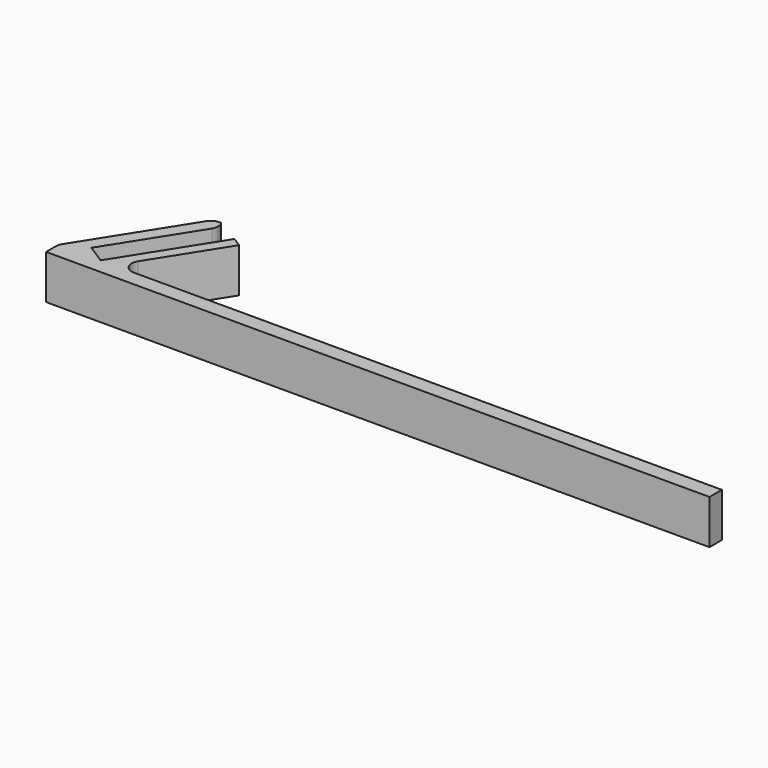
from build123d import *

# Parameters (mm, degrees)
F1_DEPTH    = 2
F2_T1_DEPTH = 2
F2_T3_DEPTH = 2.7234665539
F2_T5_DEPTH = 4.5


# Not quite as in the source:
# - a fillet or chamfer that OpenCascade refuses, or shapes differently, is made with other operations: its cross-section is extruded or revolved along the edge and cut away or added


with BuildPart() as f1:
    # F0 (on Top) → F1 (new body)
    with BuildSketch(Plane.XY):
        Polygon((0, 0.7), (0, 0), (30, 0), (30, 0.7), (2.4998066677, 0.7), (5.0013818819, 4.6602413969), (4.5786552685, 4.9272661341), (1.9084078958, 0.7), (1.0515667407, 1.2412429146), (3.7218141134, 5.4685090487), (3.2145421773, 5.7889387335), align=None)
    extrude(amount=F1_DEPTH)

    # F2: fillet of radius 0.5 on 4 edges, made by hand

    # F2_s2 → F2_t1 (join)
    with BuildSketch(Plane.XY):
        with BuildLine():
            ThreePointArc((3.4070416429, 0.7), (2.9691419006, 0.9586624445), (2.9843150295, 1.4670247373))
            Line((2.9843150295, 1.4670247373), (2.4998066677, 0.7))
            Line((2.4998066677, 0.7), (3.4070416429, 0.7))
        make_face()
    extrude(amount=F2_T1_DEPTH)

    # F2_s4 → F2_t3 (cut)
    with BuildSketch(Plane.XY.offset(-0.3617332769)):
        with BuildLine():
            ThreePointArc((0.0772733866, 0.8223314265), (0.0197067007, 0.6942971445), (0, 0.5553066892))
            Line((0, 0.5553066892), (0, 0.7))
            Line((0, 0.7), (0.0772733866, 0.8223314265))
        make_face()
    extrude(amount=F2_T3_DEPTH, mode=Mode.SUBTRACT)

    # F2_s6 → F2_t5 (cut)
    with BuildSketch(Plane.XY.offset(-1.25)):
        with BuildLine():
            ThreePointArc((3.6372687907, 5.5219139962), (3.2601462009, 5.5869152402), (2.94751744, 5.3662121201))
            Line((2.94751744, 5.3662121201), (3.2145421773, 5.7889387335))
            Line((3.2145421773, 5.7889387335), (3.6372687907, 5.5219139962))
        make_face()
        with BuildLine():
            ThreePointArc((3.4547893761, 5.0457824353), (3.5197906201, 5.4229050251), (3.2990874999, 5.735533786))
            Line((3.2990874999, 5.735533786), (3.7218141134, 5.4685090487))
            Line((3.7218141134, 5.4685090487), (3.4547893761, 5.0457824353))
        make_face()
    extrude(amount=F2_T5_DEPTH, mode=Mode.SUBTRACT)


solid = f1.part
